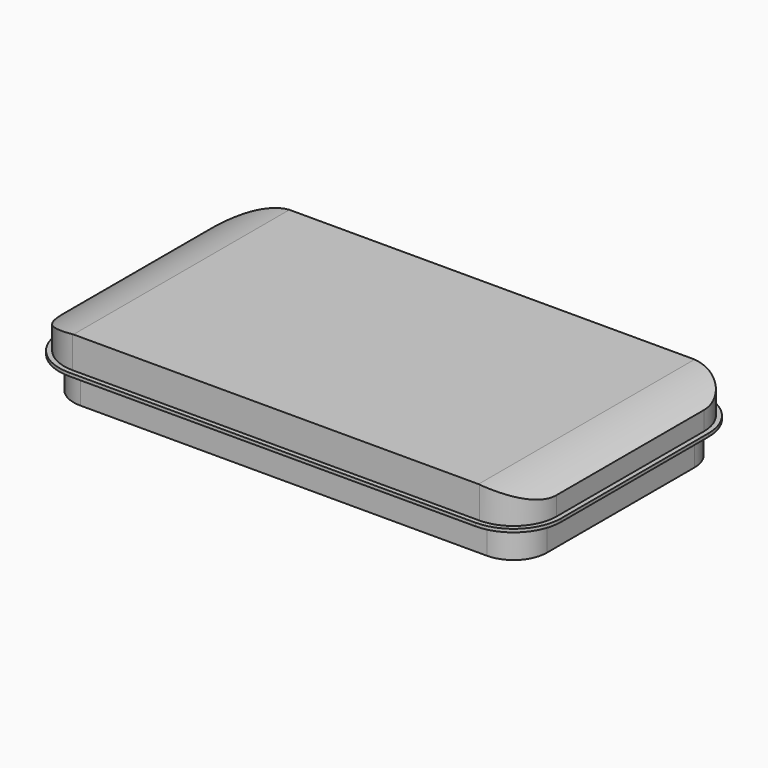
from build123d import *

# Parameters (mm, degrees)
F1_DEPTH     = 1
F2_DEPTH     = 11
F4_DEPTH     = 88.001
F5_T         = 1
F5_T3_DEPTH  = 130
F5_T5_DEPTH  = 60
F5_T8_ANGLE  = 90.000000001
F5_T10_ANGLE = 90.000000001
F5_T12_ANGLE = 90.000000001
F5_T14_ANGLE = 90.000000001
F8_DEPTH     = 10


# Not quite as in the source:
# - a shell that OpenCascade refuses in one call is made with other operations: the cavity is built on its own and cut out


with BuildPart() as f1:
    # F0 (on Top) → F1 (new body)
    with BuildSketch(Plane.XY):
        with BuildLine():
            ThreePointArc((0, 15), (4.3933982822, 4.3933982822), (15, 0))
            Line((15, 0), (143, 0))
            ThreePointArc((143, 0), (153.6066017178, 4.3933982822), (158, 15))
            Line((158, 15), (158, 73))
            ThreePointArc((158, 73), (153.6066017178, 83.6066017178), (143, 88))
            Line((143, 88), (15, 88))
            ThreePointArc((15, 88), (4.3933982822, 83.6066017178), (0, 73))
            Line((0, 73), (0, 15))
        make_face()
        with BuildLine():
            ThreePointArc((1.5, 73), (5.454058454, 82.545941546), (15, 86.5))
            Line((15, 86.5), (143, 86.5))
            ThreePointArc((143, 86.5), (152.545941546, 82.545941546), (156.5, 73))
            Line((156.5, 73), (156.5, 15))
            ThreePointArc((156.5, 15), (152.545941546, 5.454058454), (143, 1.5))
            Line((143, 1.5), (15, 1.5))
            ThreePointArc((15, 1.5), (5.454058454, 5.454058454), (1.5, 15))
            Line((1.5, 15), (1.5, 73))
        make_face(mode=Mode.SUBTRACT)
    extrude(amount=F1_DEPTH)

    # F0 (on Top) → F2 (join)
    with BuildSketch(Plane.XY):
        with BuildLine():
            Line((143, 86.5), (15, 86.5))
            ThreePointArc((15, 86.5), (5.454058454, 82.545941546), (1.5, 73))
            Line((1.5, 73), (1.5, 15))
            ThreePointArc((1.5, 15), (5.454058454, 5.454058454), (15, 1.5))
            Line((15, 1.5), (143, 1.5))
            ThreePointArc((143, 1.5), (152.545941546, 5.454058454), (156.5, 15))
            Line((156.5, 15), (156.5, 73))
            ThreePointArc((156.5, 73), (152.545941546, 82.545941546), (143, 86.5))
        make_face()
    extrude(amount=F2_DEPTH)

    # F3 (on Front) → F4 (cut, through all)
    with BuildSketch(Plane.XZ):
        with BuildLine():
            ThreePointArc((0, 6.0560618341), (7.3283980564, 9.4088283813), (15.2286913721, 11))
            ThreePointArc((15.2286913721, 11), (15.6141911349, 11.030157259), (16, 11.0560618341))
            Line((16, 11.0560618341), (0, 11.0560618341))
            Line((0, 11.0560618341), (0, 6.0560618341))
        make_face()
        with BuildLine():
            ThreePointArc((142, 11.0560618341), (142.3858088651, 11.030157259), (142.7713086279, 11))
            ThreePointArc((142.7713086279, 11), (150.6716019436, 9.4088283813), (158, 6.0560618341))
            Line((158, 6.0560618341), (158, 11.0560618341))
            Line((158, 11.0560618341), (142, 11.0560618341))
        make_face()
    extrude(amount=-F4_DEPTH, mode=Mode.SUBTRACT)

    # F5: shell of thickness 1, made by hand


with BuildPart() as f5_core1:
    # F5_t2: copy of F1
    add(f1.part)

    # the walls: a layer under each face that stays
    f5_faces = [f5_core1.faces().sort_by_distance(p)[0] for p in [
        (0, 44, 0.5),
        (4.3933982822, 83.6066017178, 0.5),
        (4.3933982822, 4.3933982822, 0.5),
        (133.3125, 1.0864197531, 1),
        (79, 88, 0.5),
        (79, 0, 0.5),
        (153.6066017178, 4.3933982822, 0.5),
        (158, 44, 0.5),
        (153.6066017178, 83.6066017178, 0.5),
        (5.454058454, 82.545941546, 5.9900432581),
        (79, 86.5, 6),
        (152.545941546, 82.545941546, 5.9900432581),
        (156.5, 44, 3.9570518678),
        (152.545941546, 5.454058454, 5.9900432581),
        (79, 1.5, 6),
        (5.454058454, 5.454058454, 5.9900432581),
        (1.5, 44, 3.9570518678),
        (8.1534990202, 44, 9.6655007895),
        (79, 44, 11),
        (149.8465009798, 44, 9.6655007895),
    ]]
    thicken(f5_faces, amount=-F5_T, mode=Mode.SUBTRACT)

    # F5_s4 → F5_t3 (cut)
    with BuildSketch(Plane.YZ.offset(14)):
        Polygon((86.51, 1.01), (86.5, 0), (85.5, 0), (85.5, 1), align=None)
        Polygon((1.49, 1.01), (1.5, 0), (2.5, 0), (2.5, 1), align=None)
    extrude(amount=F5_T3_DEPTH, mode=Mode.SUBTRACT)

    # F5_s6 → F5_t5 (cut)
    with BuildSketch(Plane.XZ.offset(-74)):
        Polygon((156.51, 1.01), (156.5, 0), (155.5, 0), (155.5, 1), align=None)
        Polygon((1.49, 1.01), (1.5, 0), (2.5, 0), (2.5, 1), align=None)
    extrude(amount=F5_T5_DEPTH, mode=Mode.SUBTRACT)

    # F5_s7 → F5_t8 (revolve, cut)
    with BuildSketch(Plane.XZ.offset(-73)):
        Polygon((1.49, 1.01), (1.5, 0), (2.5, 0), (2.5, 1), align=None)
    revolve(axis=Axis((15, 73, 1), (0, 0, -1)), revolution_arc=F5_T8_ANGLE, mode=Mode.SUBTRACT)

    # F5_s9 → F5_t10 (revolve, cut)
    with BuildSketch(Plane.YZ.offset(143)):
        Polygon((86.51, 1.01), (86.5, 0), (85.5, 0), (85.5, 1), align=None)
    revolve(axis=Axis((143, 73, 1), (0, 0, -1)), revolution_arc=F5_T10_ANGLE, mode=Mode.SUBTRACT)

    # F5_s11 → F5_t12 (revolve, cut)
    with BuildSketch(Plane.XZ.offset(-15)):
        Polygon((156.51, 1.01), (156.5, 0), (155.5, 0), (155.5, 1), align=None)
    revolve(axis=Axis((143, 15, 1), (0, 0, -1)), revolution_arc=F5_T12_ANGLE, mode=Mode.SUBTRACT)

    # F5_s13 → F5_t14 (revolve, cut)
    with BuildSketch(Plane.YZ.offset(15)):
        Polygon((1.49, 1.01), (1.5, 0), (2.5, 0), (2.5, 1), align=None)
    revolve(axis=Axis((15, 15, 1), (0, 0, -1)), revolution_arc=F5_T14_ANGLE, mode=Mode.SUBTRACT)


with BuildPart() as f1_1:
    add(f1.part)

    # what is left inside the walls is the cavity
    f5_cavity = [f5_core1.part.solids().sort_by_distance(p)[0] for p in [
        (79, 30.166667, 0.01),
    ]]
    add(f5_cavity, mode=Mode.SUBTRACT)

    # F6 (on Top) → F7 (join, up to the next surface of F1)
    with BuildSketch(Plane.XY):
        with BuildLine():
            Line((143, 83.5), (15, 83.5))
            ThreePointArc((15, 83.5), (7.5753787975, 80.4246212025), (4.5, 73))
            Line((4.5000000324, 73), (4.5000000324, 14.9847623929))
            ThreePointArc((4.5000000324, 14.9847623929), (7.5753788898, 7.5753631149), (14.9847847018, 4.5))
            Line((14.9847847018, 4.5), (143, 4.5))
            ThreePointArc((143, 4.5), (150.4246212025, 7.5753787975), (153.5, 15))
            Line((153.5, 15), (153.5, 73))
            ThreePointArc((153.5, 73), (150.4246212025, 80.4246212025), (143, 83.5))
        make_face()
    extrude(until=Until.NEXT)

    # F6 (on Top) → F8 (join)
    with BuildSketch(Plane.XY):
        with BuildLine():
            Line((143, 83.5), (15, 83.5))
            ThreePointArc((15, 83.5), (7.5753787975, 80.4246212025), (4.5, 73))
            Line((4.5000000324, 73), (4.5000000324, 14.9847623929))
            ThreePointArc((4.5000000324, 14.9847623929), (7.5753788898, 7.5753631149), (14.9847847018, 4.5))
            Line((14.9847847018, 4.5), (143, 4.5))
            ThreePointArc((143, 4.5), (150.4246212025, 7.5753787975), (153.5, 15))
            Line((153.5, 15), (153.5, 73))
            ThreePointArc((153.5, 73), (150.4246212025, 80.4246212025), (143, 83.5))
        make_face()
    extrude(amount=-F8_DEPTH)


solid = f1_1.part
